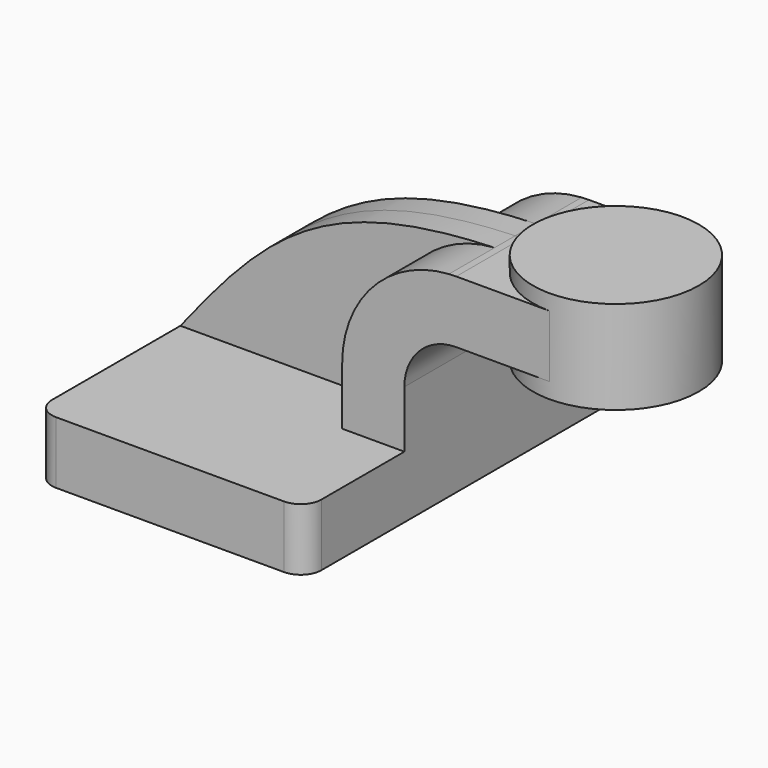
from build123d import *

# Parameters (mm, degrees)
F1_DEPTH = 63.5
F2_DEPTH = 25.4
F3_DEPTH = 7.9375
F0_W     = 25.4
F0_H     = 19.05
F4_DEPTH = 25.4
F6_R     = 6.35


with BuildPart() as f1:
    # F0 (on Front) → F1 (new body, symmetric)
    with BuildSketch(Plane.XZ):
        Polygon((22.225, 9.525), (-41.275, 9.525), (-41.275, -9.525), (41.275, -9.525), (41.275, 9.525), align=None)
    extrude(amount=F1_DEPTH, both=True)

    # F0 (on Front) → F2 (join, symmetric)
    with BuildSketch(Plane.XZ):
        with BuildLine():
            Line((22.225, 27.0002), (22.225, 9.525))
            Line((22.225, 9.525), (41.275, 9.525))
            Line((41.275, 9.525), (41.275, 27.0002))
            ThreePointArc((41.275, 27.0002), (45.9246798487, 38.2255201513), (57.15, 42.8752))
            Line((57.15, 42.8752), (60.325, 42.8752))
            Line((60.325, 42.8752), (60.325, 61.9252))
            Line((60.325, 61.9252), (57.15, 61.9252))
            add(Edge.make_bspline(
                [(54.9309637921, 61.854633051), (55.6637542078, 61.8810124388), (56.4033914289, 61.9045304692), (57.15, 61.9252)],
                knots=[109.9388089339, 109.9388089339, 109.9388089339, 109.9388089339, 111.5045361635, 111.5045361635, 111.5045361635, 111.5045361635], degree=3))
            ThreePointArc((54.9309637921, 61.854633051), (31.6818290354, 50.8984822127), (22.225, 27.0002))
        make_face()
    extrude(amount=F2_DEPTH, both=True)

    # F0 (on Front) → F3 (join, symmetric)
    with BuildSketch(Plane.XZ):
        with BuildLine():
            add(Edge.make_bspline(
                [(-41.275, 9.525), (-14.2194517609, 44.0428960459), (3.4774896668, 60.0023829163), (54.9309637921, 61.854633051)],
                knots=[0, 0, 0, 0, 109.9388089339, 109.9388089339, 109.9388089339, 109.9388089339], degree=3))
            Line((-41.275, 9.525), (22.225, 9.525))
            Line((22.225, 9.525), (22.225, 27.0002))
            ThreePointArc((22.225, 27.0002), (31.6818290354, 50.8984822127), (54.9309637921, 61.854633051))
        make_face()
    extrude(amount=F3_DEPTH, both=True)

    # F0 (on Front) → F4 (join, symmetric)
    with BuildSketch(Plane.XZ):
        with Locations((73.025, 52.4002)):
            Rectangle(F0_W, F0_H)
    extrude(amount=F4_DEPTH, both=True)

    # F0 (on Front) → F5 (revolve)
    with BuildSketch(Plane.XZ):
        Polygon((85.725, 66.675), (85.725, 61.9252), (85.725, 42.8752), (85.725, 38.1), (111.125, 38.1), (111.125, 66.675), align=None)
    revolve(axis=Axis((85.725, 0, 52.3875), (0, 0, 1)))

    # F6
    f6_edges = [f1.edges().sort_by_distance(p)[0] for p in [
        (41.275, -63.5, 0),
        (-41.275, -63.5, 0),
        (41.275, 63.5, 0),
        (-41.275, 63.5, 0),
    ]]
    fillet(f6_edges, radius=F6_R)


solid = f1.part
